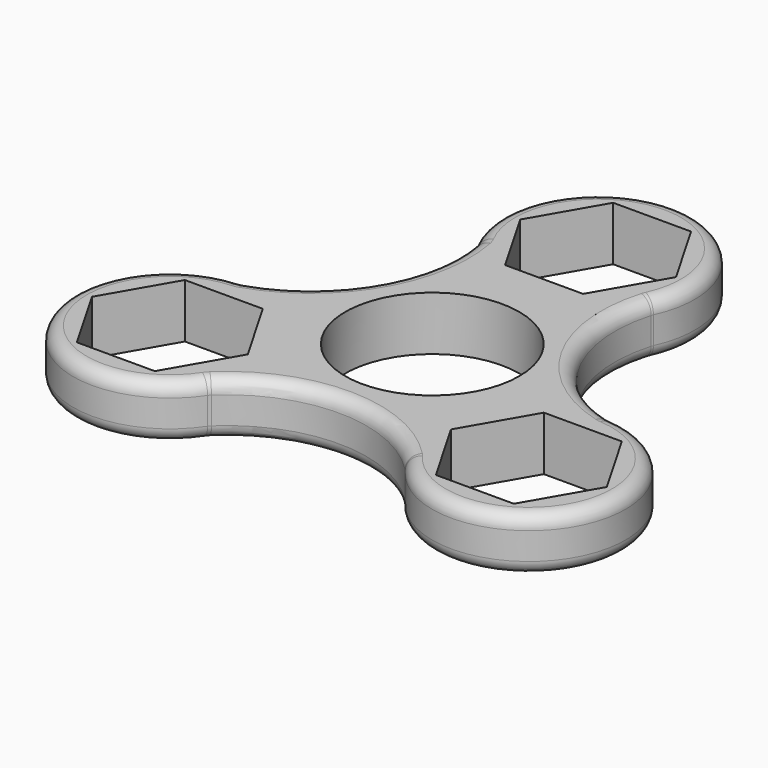
from build123d import *

# Parameters (mm, degrees)
F0_R     = 11.25
F1_DEPTH = 7
F2_F1_R  = 1.75
F2_F2_R  = 1.75


# Not quite as in the source:
# - a feature names something its author has since deleted; it is built from what else it names


with BuildPart() as f1:
    # F0 (on Top) → F1 (new body)
    with BuildSketch(Plane.XY):
        with BuildLine():
            ThreePointArc((23.8479882297, -0.9143272054), (12.8207682574, 7.5970822448), (11.2961561087, 21.4433535458))
            ThreePointArc((11.2961561087, 21.4433535458), (-0.3696422444, 39.2901628216), (-10.9599899611, 20.7849206513))
            ThreePointArc((-10.9599899611, 20.7849206513), (-13.1426262864, 7.4651290037), (-23.7284148542, -0.908748907))
            ThreePointArc((-23.7284148542, -0.908748907), (-34.0498321112, -19.6151057374), (-12.6918356784, -20.1586390273))
            ThreePointArc((-12.6918356784, -20.1586390273), (0.2517315357, -15.0201868131), (13.0027753206, -20.6193390506))
            ThreePointArc((13.0027753206, -20.6193390506), (34.1566443936, -19.4249802921), (23.8479882297, -0.9143272054))
        make_face()
        Polygon((-13.1309336016, -13.3978147163), (-18.1683147003, -22.1228147163), (-28.2430768977, -22.1228147163), (-33.2804579963, -13.3978147163), (-28.2430768977, -4.6728147163), (-18.1683147003, -4.6728147163), align=None, mode=Mode.SUBTRACT)
        Polygon((18.1683147003, -4.6728147163), (28.2430768977, -4.6728147163), (33.2804579963, -13.3978147163), (28.2430768977, -22.1228147163), (18.1683147003, -22.1228147163), (13.1309336016, -13.3978147163), align=None, mode=Mode.SUBTRACT)
        Circle(F0_R, mode=Mode.SUBTRACT)
        Polygon((-5.0373810987, 35.5206294325), (5.0373810987, 35.5206294325), (10.0747621974, 26.7956294325), (5.0373810987, 18.0706294325), (-5.0373810987, 18.0706294325), (-10.0747621974, 26.7956294325), align=None, mode=Mode.SUBTRACT)
    extrude(amount=F1_DEPTH)

    # F2: fillet of radius 1.75 on 14 edges, made by hand

    # F2_f1
    f2_f1_edges = [f1.edges().sort_by_distance(p)[0] for p in [
        (13.0027753206, -20.6193390506, 3.5),
        (23.8479882297, -0.9143272054, 3.5),
        (11.2961561087, 21.4433535458, 3.5),
        (-10.9599899611, 20.7849206513, 3.5),
        (-23.7284148542, -0.908748907, 3.5),
        (-12.6918356784, -20.1586390273, 3.5),
    ]]
    fillet(f2_f1_edges, radius=F2_F1_R)

    # F2_f2
    f2_f2_edges = [f1.edges().sort_by_distance(p)[0] for p in [
        (-34.043255935, -19.6265618053, 0),
        (-34.043255935, -19.6265618053, 7),
        (-23.7183868319, -0.8923048018, 7),
        (-12.6760959015, -20.1569074189, 7),
        (-23.7183868319, -0.8923048018, 0),
        (-12.6760959015, -20.1569074189, 0),
    ]]
    fillet(f2_f2_edges, radius=F2_F2_R)


solid = f1.part
